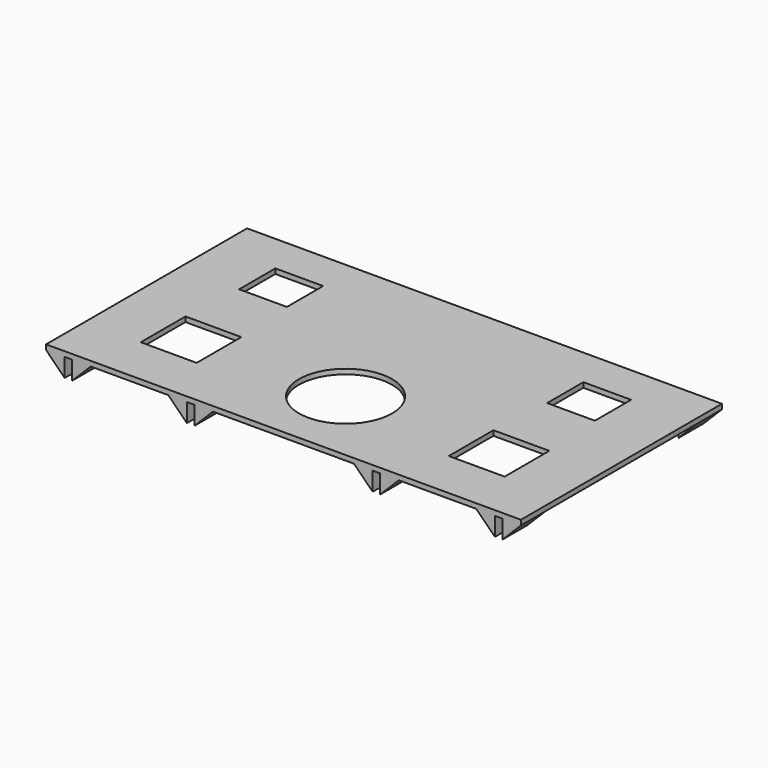
from build123d import *

# Parameters (mm, degrees)
F2_DEPTH  = 81
F3_DEPTH  = 10
F4_START  = -71
F4_DEPTH  = 10
F8_R      = 15
F9_DEPTH  = 1.6
F10_W     = 15.4
F10_H     = 14.6
F11_DEPTH = 1.6
F12_W     = 18
F12_H     = 18
F13_DEPTH = 1.6


# Not quite as in the source:
# - a feature names something its author has since deleted; it is built from what else it names


with BuildPart() as f2:
    # F1 (on offset) → F2 (new body)
    with BuildSketch(Plane.XZ.offset(40.5)):
        Polygon((76.55, 0), (76.55, 1.6), (-76.55, 1.6), (-76.55, 0), (-70.55, 0), (-68.15, 0), (-62.15, 0), (-37.15, 0), (-31.15, 0), (-28.75, 0), (-22.75, 0), (22.75, 0), (28.75, 0), (31.15, 0), (37.15, 0), (62.15, 0), (68.15, 0), (70.55, 0), align=None)
    extrude(amount=-F2_DEPTH)

    # F1 (on offset) → F3 (join)
    with BuildSketch(Plane.XZ.offset(40.5)):
        Polygon((-62.15, 0), (-68.15, 0), (-68.15, -6), align=None)
        Polygon((-31.15, 0), (-37.15, 0), (-31.15, -6), align=None)
        Polygon((-22.75, 0), (-28.75, 0), (-28.75, -6), align=None)
        Polygon((-70.55, 0), (-76.55, 0), (-70.55, -6), align=None)
    extrude(amount=-F3_DEPTH)

    # F1 (on offset) → F4 (join)
    with BuildSketch(Plane.XZ.offset(40.5).offset(F4_START)):
        Polygon((-62.15, 0), (-68.15, 0), (-68.15, -6), align=None)
        Polygon((-31.15, 0), (-37.15, 0), (-31.15, -6), align=None)
        Polygon((-22.75, 0), (-28.75, 0), (-28.75, -6), align=None)
        Polygon((-70.55, 0), (-76.55, 0), (-70.55, -6), align=None)
    extrude(amount=-F4_DEPTH)

    # F7: F2 across plane


with BuildPart() as f2_1:
    add(f2.part)
    add(f2.part.mirror(Plane.YZ))

    # F8 (on face) → F9 (cut)
    with BuildSketch(Plane.XY.offset(1.6)):
        with Locations((0, -15.5)):
            Circle(F8_R)
    extrude(amount=-F9_DEPTH, mode=Mode.SUBTRACT)

    # F10 (on face) → F11 (cut)
    with BuildSketch(Plane.XY.offset(1.6)):
        with Locations((-49.65, 20.6)):
            Rectangle(F10_W, F10_H)
        with Locations((49.65, 20.6)):
            Rectangle(F10_W, F10_H)
    extrude(amount=-F11_DEPTH, mode=Mode.SUBTRACT)

    # F12 (on Top) → F13 (cut)
    with BuildSketch(Plane.XY):
        with Locations((-49.65, -15.7)):
            Rectangle(F12_W, F12_H)
        with Locations((49.65, -15.7)):
            Rectangle(F12_W, F12_H)
    extrude(amount=F13_DEPTH, mode=Mode.SUBTRACT)


solid = f2_1.part
